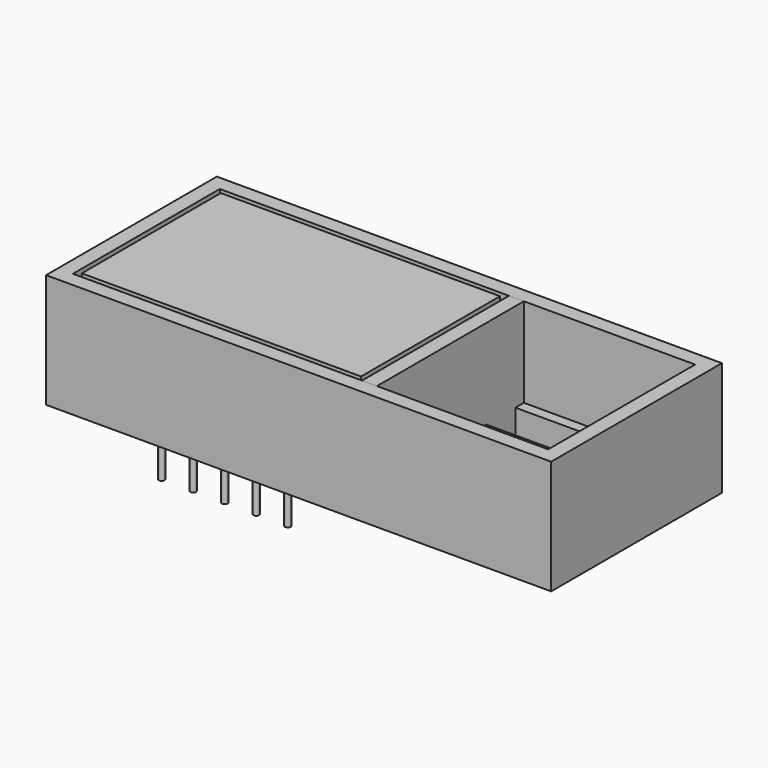
from build123d import *

# Parameters (mm, degrees)
F4_W      = 22.5
F4_H      = 14
F6_DEPTH  = 6.2
F5_R      = 0.225
F7_DEPTH  = 7.6
F10_DEPTH = 14
F11_W     = 25.7
F11_H     = 17.2
F11_W_2   = 23.3
F11_H_2   = 14.8
F12_DEPTH = 7.2
F11_W_3   = 13.1
F11_H_3   = 2.94
F11_W_4   = 15.64
F13_DEPTH = 2
F14_W     = 40.7
F14_H     = 17.2
F14_W_2   = 38.3
F14_H_2   = 14.8
F15_DEPTH = 7.2
F14_W_3   = 13.1
F14_H_3   = 2.94
F14_W_4   = 15.64
F16_DEPTH = 2


# Not quite as in the source:
# - a feature names something its author has since deleted; it is built from what else it names


with BuildPart() as f6:
    # F4 (on offset) → F6 (new body, through all)
    with BuildSketch(Plane.XY.offset(7.2)):
        with Locations((-95.4044193358, 19.5834040642)):
            Rectangle(F4_W, F4_H)
    extrude(amount=-F6_DEPTH)

    # F5 (on offset) → F7 (join, through all)
    with BuildSketch(Plane.XY.offset(1)):
        with Locations((-91.5944193358, 24.6634040642)):
            Circle(F5_R)
        with Locations((-94.1344193358, 24.6634040642)):
            Circle(F5_R)
        with Locations((-96.6744193358, 24.6634040642)):
            Circle(F5_R)
        with Locations((-99.2144193358, 24.6634040642)):
            Circle(F5_R)
        with Locations((-101.7544193358, 24.6634040642)):
            Circle(F5_R)
        with Locations((-101.7544193358, 14.5034040642)):
            Circle(F5_R)
        with Locations((-99.2144193358, 14.5034040642)):
            Circle(F5_R)
        with Locations((-96.6744193358, 14.5034040642)):
            Circle(F5_R)
        with Locations((-94.1344193358, 14.5034040642)):
            Circle(F5_R)
        with Locations((-91.5944193358, 14.5034040642)):
            Circle(F5_R)
        with Locations((-89.0544193358, 24.6634040642)):
            Circle(F5_R)
    extrude(amount=-F7_DEPTH)

    # F9 (on offset) → F10 (join, through all)
    with BuildSketch(Plane.XZ.offset(-12.5834040642)):
        Polygon((-104.6495500536, 1), (-106.6544193358, 1), (-106.6544193358, 0), (-105.420655343, 0), align=None)
        Polygon((-86.1592886181, 1), (-85.3881833286, 0), (-84.1544193358, 0), (-84.1544193358, 1), align=None)
    extrude(amount=-F10_DEPTH)


with BuildPart() as f12:
    # F11 (on offset) → F12 (new body, through all)
    with BuildSketch(Plane.XY):
        with Locations((-95.4044193358, 19.5834040642)):
            Rectangle(F11_W, F11_H)
        with Locations((-95.4044193358, 19.5834040642)):
            Rectangle(F11_W_2, F11_H_2, mode=Mode.SUBTRACT)
    extrude(amount=F12_DEPTH)

    # F11 (on offset) → F13 (join)
    with BuildSketch(Plane.XY):
        with Locations((-95.4044193358, 19.5834040642)):
            Rectangle(F11_W, F11_H)
        with Locations((-95.4044193358, 19.5834040642)):
            Rectangle(F11_W_2, F11_H_2, mode=Mode.SUBTRACT)
        with Locations((-95.4044193358, 19.5834040642)):
            Rectangle(F11_W_2, F11_H_2)
        with Locations((-96.6744193358, 14.5034040642)):
            Rectangle(F11_W_3, F11_H_3, mode=Mode.SUBTRACT)
        with Locations((-95.4044193358, 24.6634040642)):
            Rectangle(F11_W_4, F11_H_3, mode=Mode.SUBTRACT)
    extrude(amount=-F13_DEPTH)


with BuildPart() as f15:
    # F14 (on offset) → F15 (new body, through all)
    with BuildSketch(Plane.XY):
        with Locations((-87.9044193358, 19.5834040642)):
            Rectangle(F14_W, F14_H)
        with Locations((-87.9044193358, 19.5834040642)):
            Rectangle(F14_W_2, F14_H_2, mode=Mode.SUBTRACT)
    extrude(amount=F15_DEPTH)

    # F14 (on offset) → F16 (join)
    with BuildSketch(Plane.XY):
        with Locations((-87.9044193358, 19.5834040642)):
            Rectangle(F14_W, F14_H)
        with Locations((-87.9044193358, 19.5834040642)):
            Rectangle(F14_W_2, F14_H_2, mode=Mode.SUBTRACT)
        with Locations((-87.9044193358, 19.5834040642)):
            Rectangle(F14_W_2, F14_H_2)
        with Locations((-96.6744193358, 14.5034040642)):
            Rectangle(F14_W_3, F14_H_3, mode=Mode.SUBTRACT)
        with Locations((-76.2544193358, 14.5034040642)):
            Rectangle(F14_W_3, F14_H_3, mode=Mode.SUBTRACT)
        with Locations((-95.4044193358, 24.6634040642)):
            Rectangle(F14_W_4, F14_H_3, mode=Mode.SUBTRACT)
        with Locations((-76.2544193358, 24.6634040642)):
            Rectangle(F14_W_3, F14_H_3, mode=Mode.SUBTRACT)
    extrude(amount=-F16_DEPTH)


solid = Compound([f6.part, f12.part, f15.part])
